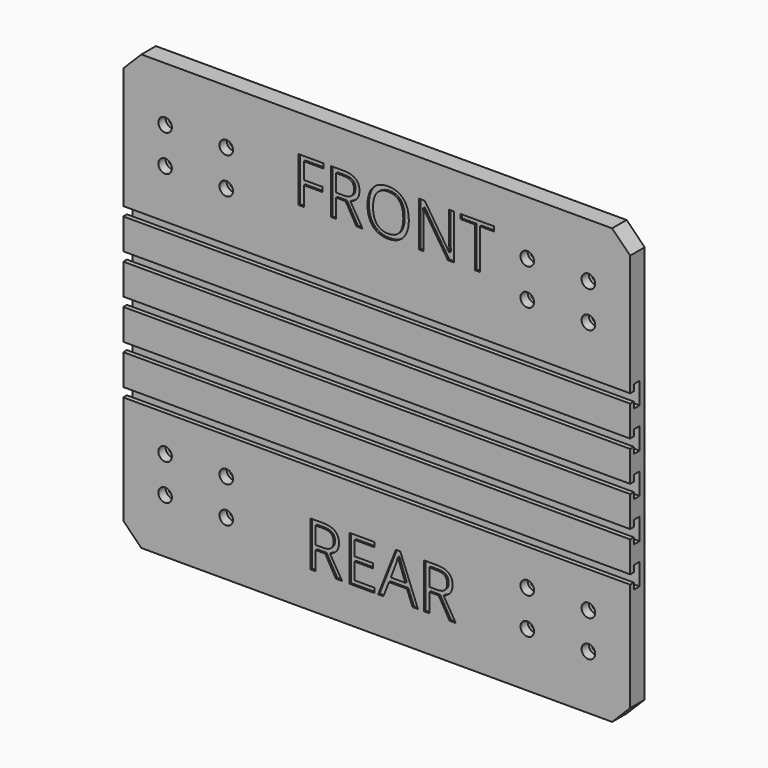
from build123d import *

# Parameters (mm, degrees)
F0_W           = 355.6
F0_H           = 304.8
F1_DEPTH       = 12.7
F4_D           = 4.7752
F4_CBORE_D     = 9.525
F4_CBORE_DEPTH = 6.35
F6_DEPTH       = 355.601
F7_TEXT_SIZE   = 44.0972222222
F8_DEPTH       = 1.27
F9_TEXT_SIZE   = 44.0972222222
F10_DEPTH      = 1.27
F12_D          = 6.35
F12_DEPTH      = 6.35
F12_TIP        = 1.9077324654
F13_SIZE       = 12.7


# Not quite as in the source:
# - Text() gives the source's letters only with a copy of the font that has no kerning and outlines rounded to 1/6400 em; it was checked with that copy


with BuildPart() as f1:
    # F0 (on Front) → F1 (new body)
    with BuildSketch(Plane.XZ):
        with Locations((177.8, 152.4)):
            Rectangle(F0_W, F0_H)
    extrude(amount=F1_DEPTH)

    # F4 (through all)
    with Locations(Plane.XZ.offset(12.7)):
        with Locations((29.337, 266.7), (72.2122, 266.7), (72.2122, 241.3), (29.337, 241.3), (29.337, 63.5), (72.2122, 63.5), (72.2122, 38.1), (29.337, 38.1), (283.3624, 38.1), (283.3624, 63.5), (326.2376, 63.5), (326.2376, 38.1), (283.3624, 241.3), (326.2376, 241.3), (326.2376, 266.7), (283.3624, 266.7)):
            CounterBoreHole(F4_D / 2, F4_CBORE_D / 2, F4_CBORE_DEPTH)

    # F5 (on face) → F6 (cut, through all)
    with BuildSketch(Plane.YZ.offset(355.6)):
        Polygon((-9.525, 151.13), (-12.7, 151.13), (-12.7, 144.78), (-9.525, 144.78), (-9.525, 140.335), (-4.445, 140.335), (-4.445, 155.575), (-9.525, 155.575), align=None)
        Polygon((-9.525, 179.07), (-12.7, 179.07), (-12.7, 172.72), (-9.525, 172.72), (-9.525, 168.275), (-4.445, 168.275), (-4.445, 183.515), (-9.525, 183.515), align=None)
        Polygon((-9.525, 207.01), (-12.7, 207.01), (-12.7, 200.66), (-9.525, 200.66), (-9.525, 196.215), (-4.445, 196.215), (-4.445, 211.455), (-9.525, 211.455), align=None)
        Polygon((-12.7, 123.19), (-12.7, 116.84), (-9.525, 116.84), (-9.525, 112.395), (-4.445, 112.395), (-4.445, 127.635), (-9.525, 127.635), (-9.525, 123.19), align=None)
        Polygon((-12.7, 95.25), (-12.7, 88.9), (-9.525, 88.9), (-9.525, 84.455), (-4.445, 84.455), (-4.445, 99.695), (-9.525, 99.695), (-9.525, 95.25), align=None)
    extrude(amount=-F6_DEPTH, mode=Mode.SUBTRACT)

    # F7 (on face) → F8 (cut)
    with BuildSketch(Plane.XZ.offset(12.7)):
        with Locations((118.618, 247.65)):
            Text('FRONT', F7_TEXT_SIZE, font='Open Sans', text_align=(TextAlign.LEFT, TextAlign.BOTTOM))
    extrude(amount=-F8_DEPTH, mode=Mode.SUBTRACT)

    # F9 (on face) → F10 (cut)
    with BuildSketch(Plane.XZ.offset(12.7)):
        with Locations((127, 25.4)):
            Text('REAR', F9_TEXT_SIZE, font='Open Sans', text_align=(TextAlign.LEFT, TextAlign.BOTTOM))
    extrude(amount=-F10_DEPTH, mode=Mode.SUBTRACT)

    # F12
    with Locations(Plane(origin=(0, 0, 0), x_dir=(-1, 0, 0), z_dir=(0, 1, 0))):
        with Locations((-215.9, 101.6), (-215.9, 33.401), (-139.7, 33.401), (-139.7, 101.6)):
            Hole(F12_D / 2, depth=F12_DEPTH)
            with Locations((0, 0, -(F12_DEPTH + F12_TIP / 2))):  # 118° drill point
                Cone(0, F12_D / 2, F12_TIP, mode=Mode.SUBTRACT)

    # F13
    f13_edges = [f1.edges().sort_by_distance(p)[0] for p in [
        (0, -6.35, 304.8),
        (0, -6.35, 0),
        (355.6, -6.35, 0),
        (355.6, -6.35, 304.8),
    ]]
    chamfer(f13_edges, length=F13_SIZE)


solid = f1.part
